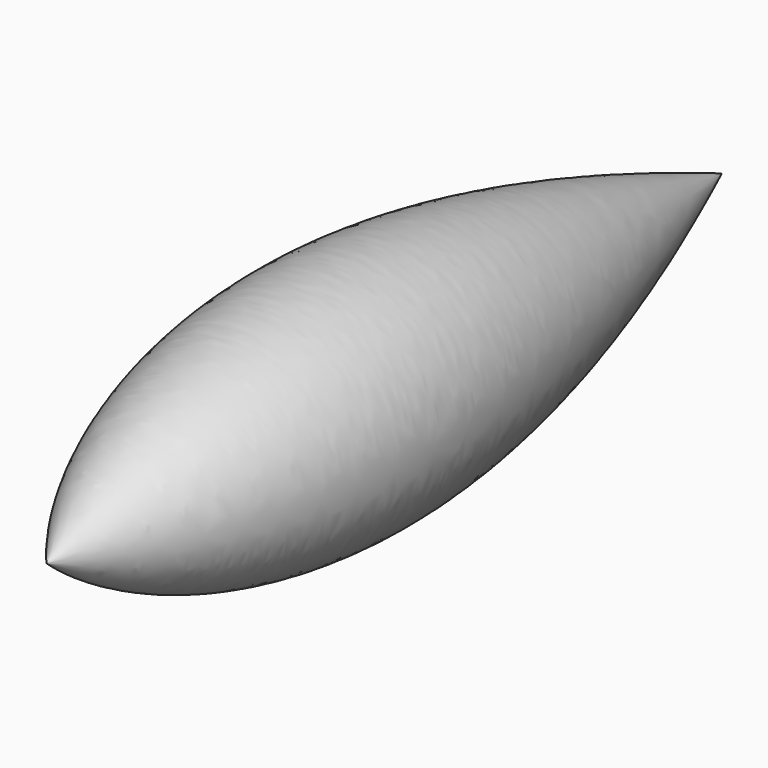
from build123d import *


with BuildPart() as f1:
    # F0 (on Top) → F1 (revolve)
    with BuildSketch(Plane.XY):
        with BuildLine():
            Line((0, 279.1217575701), (0, -170.8782424299))
            add(Edge.make_bspline(
                [(0, -170.8782424299), (39.0136756109, -125.7633686772), (82.5304449912, 10.5299481508), (43.9741604202, 171.5134214993), (0, 279.1217575701)],
                knots=[0, 0, 0, 0, 0.4435503729, 1, 1, 1, 1], degree=3))
        make_face()
    revolve(axis=Axis((0, 54.1217575701, 0), (0, 1, 0)))


solid = f1.part
